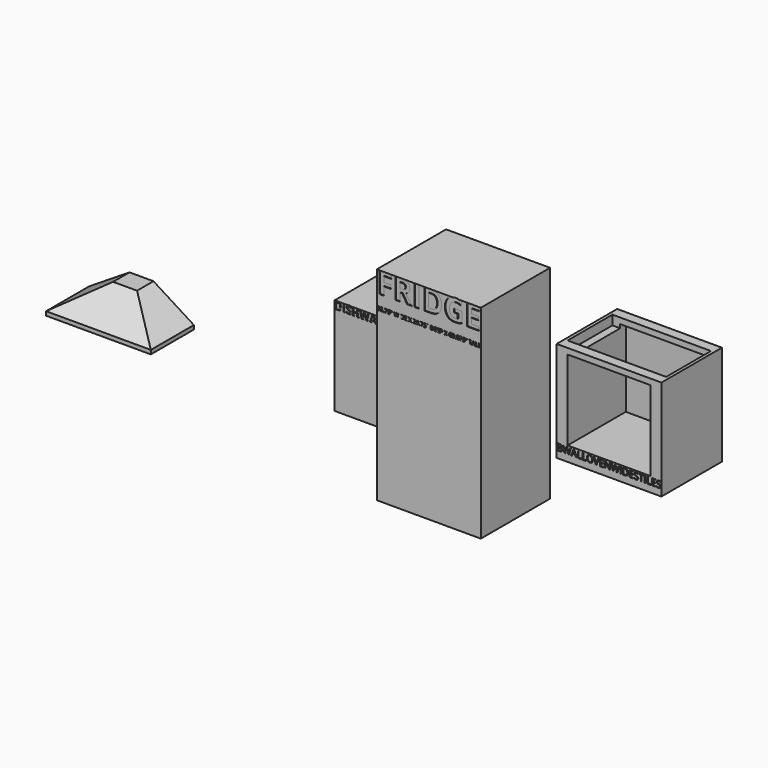
from build123d import *

# Parameters (mm, degrees)
F0_W          = 908.05
F0_H          = 755.65
F1_DEPTH      = 1774.825
F2_TEXT_SIZE  = 254.3334792123
F3_DEPTH      = 6.35
F4_W          = 609.6
F4_H          = 660.4
F5_DEPTH      = 850.9
F6_TEXT_SIZE  = 91.7359919114
F7_DEPTH      = 6.35
F8_W          = 914.4
F8_H          = 660.4
F9_DEPTH      = 876.3
F10_W         = 914.4
F10_H         = 469.9
F11_DEPTH     = 34.925
F12_W         = 914.4
F12_H         = 469.9
F14_W         = 209.55
F14_H         = 179.3875
F16_TEXT_SIZE = 46.3154203559
F17_DEPTH     = 25.4
F18_TEXT_SIZE = 79.9289782428
F19_DEPTH     = 25.4
F20_W         = 860.425
F20_H         = 488.95
F21_DEPTH     = 82.55
F22_W         = 723.9
F22_H         = 698.5
F23_DEPTH     = 635


# Not quite as in the source:
# - Text() gives the source's letters only with a copy of the font that has no kerning and outlines rounded to 1/6400 em; it was checked with that copy


with BuildPart() as f1:
    # F0 (on Top) → F1 (new body)
    with BuildSketch(Plane.XY):
        with Locations((454.025, -377.825)):
            Rectangle(F0_W, F0_H)
    extrude(amount=F1_DEPTH)

    # F2 (on face) → F3 (cut)
    with BuildSketch(Plane.XZ.offset(755.65)):
        with Locations((0, 1591.7048949672)):
            Text('FRIDGE', F2_TEXT_SIZE, font='Open Sans', font_style=FontStyle.BOLD, text_align=(TextAlign.LEFT, TextAlign.BOTTOM))
    extrude(amount=-F3_DEPTH, mode=Mode.SUBTRACT)

    # F16 (on face) → F17 (cut)
    with BuildSketch(Plane.XZ.offset(755.65)):
        with Locations((0, 1464.3302145653)):
            Text('35.75" WIDE X 29.75" DEEP X 69.875" TALL', F16_TEXT_SIZE, font='Open Sans', text_align=(TextAlign.LEFT, TextAlign.BOTTOM))
    extrude(amount=-F17_DEPTH, mode=Mode.SUBTRACT)


with BuildPart() as f5:
    # F4 (on Top) → F5 (new body)
    with BuildSketch(Plane.XY):
        with Locations((-742.6245548248, 424.0554736137)):
            Rectangle(F4_W, F4_H)
    extrude(amount=F5_DEPTH)

    # F6 (on face) → F7 (cut)
    with BuildSketch(Plane.XZ.offset(-93.8554736137)):
        with Locations((-1047.4245548248, 784.8500858238)):
            Text('DISHWASHER', F6_TEXT_SIZE, font='Open Sans', font_style=FontStyle.BOLD, text_align=(TextAlign.LEFT, TextAlign.BOTTOM))
    extrude(amount=-F7_DEPTH, mode=Mode.SUBTRACT)


with BuildPart() as f9:
    # F8 (on Top) → F9 (new body)
    with BuildSketch(Plane.XY):
        with Locations((1024.089308691, 828.6163907405)):
            Rectangle(F8_W, F8_H)
    extrude(amount=F9_DEPTH)

    # F18 (on face) → F19 (cut)
    with BuildSketch(Plane.XZ.offset(-498.4163907405)):
        with Locations((566.889308691, 58.7518492838)):
            Text('BWALLOVENWIDESTILES', F18_TEXT_SIZE, font='Open Sans', text_align=(TextAlign.LEFT, TextAlign.BOTTOM))
    extrude(amount=-F19_DEPTH, mode=Mode.SUBTRACT)

    # F20 (on face) → F21 (cut)
    with BuildSketch(Plane.XY.offset(876.3)):
        with Locations((1024.089308691, 828.6163907405)):
            Rectangle(F20_W, F20_H)
    extrude(amount=-F21_DEPTH, mode=Mode.SUBTRACT)

    # F22 (on face) → F23 (cut)
    with BuildSketch(Plane.XZ.offset(-498.4163907405)):
        with Locations((1024.089308691, 476.25)):
            Rectangle(F22_W, F22_H)
    extrude(amount=-F23_DEPTH, mode=Mode.SUBTRACT)


with BuildPart() as f11:
    # F10 (on Top) → F11 (new body)
    with BuildSketch(Plane.XY):
        with Locations((-3004.983484745, 197.8222084337)):
            Rectangle(F10_W, F10_H)
    extrude(amount=F11_DEPTH)

    # F12 (on face) → F15 section 0
    with BuildSketch(Plane.XY.offset(34.925)):
        with Locations((-3004.983484745, 197.8222084337)):
            Rectangle(F12_W, F12_H)
    # F14 (on offset) → F15 section 1
    with BuildSketch(Plane.XY.offset(257.175)):
        with Locations((-3004.983484745, 343.0784584337)):
            Rectangle(F14_W, F14_H)
    loft()


solid = Compound([f1.part, f5.part, f9.part, f11.part])
